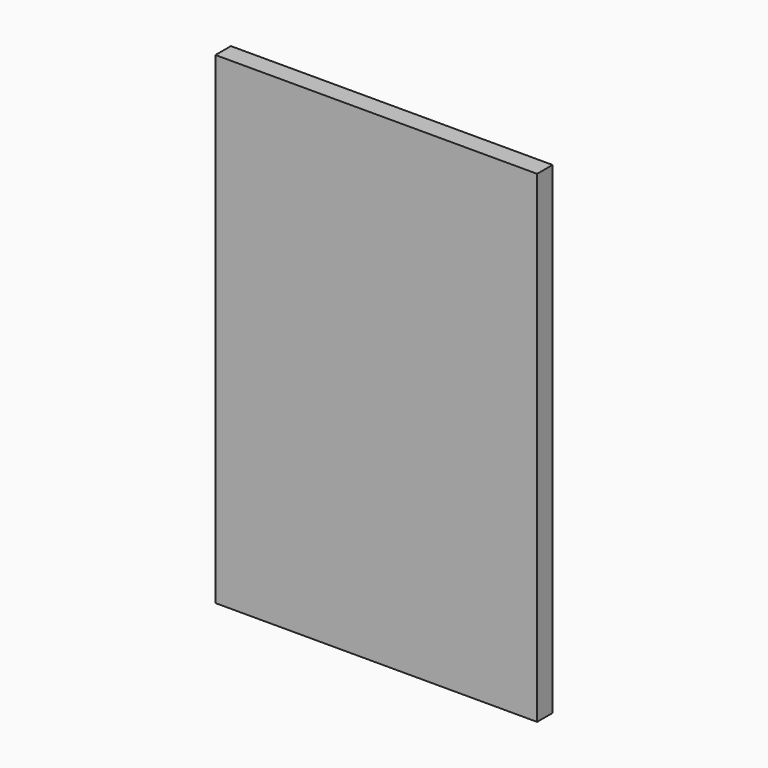
from build123d import *

# Parameters (mm, degrees)
F1_E0_TOP_W = 300
F1_E0_TOP_H = 450
F2_DEPTH    = 18


with BuildPart() as f2:
    # F1_E0_top (on explicit) → F2 (new body)
    with BuildSketch(Plane(origin=(-150, 150, 0), x_dir=(1, 0, 0), z_dir=(0, -1, 0))):
        with Locations((150, 225)):
            Rectangle(F1_E0_TOP_W, F1_E0_TOP_H)
    extrude(amount=F2_DEPTH)


solid = f2.part
